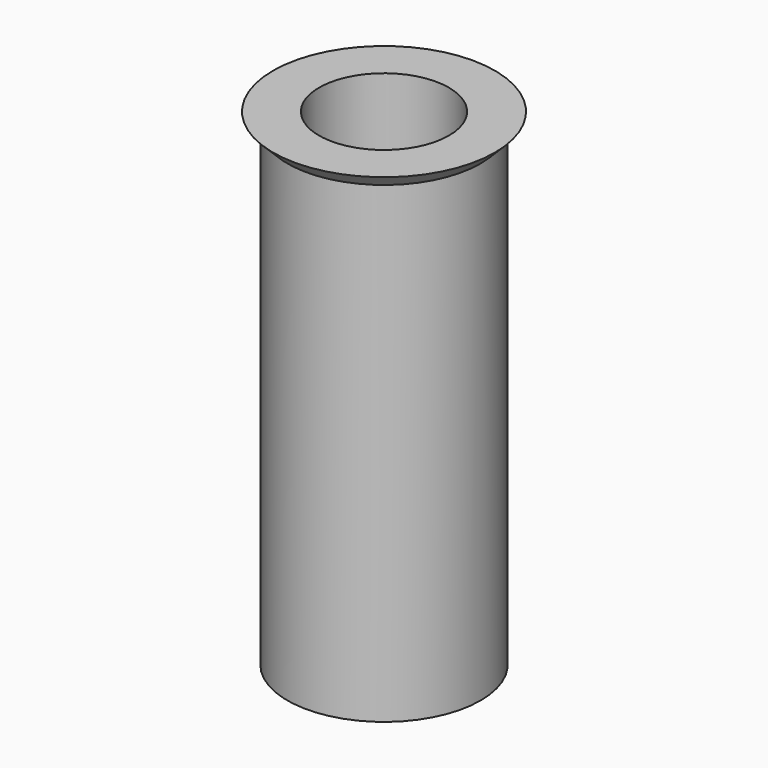
from build123d import *

# Parameters (mm, degrees)
F0_R        = 8.925
F1_DEPTH    = 45
F2_R        = 6
F3_DEPTH    = 40
F4_R        = 10.25
F4_R_2      = 8.925
F5_DEPTH    = 1.5
F6_S5_R     = 8.925
F6_T6_DEPTH = 16


# Not quite as in the source:
# - a fillet or chamfer that OpenCascade refuses, or shapes differently, is made with other operations: its cross-section is extruded or revolved along the edge and cut away or added


with BuildPart() as f1:
    # F0 (on Top) → F1 (new body)
    with BuildSketch(Plane.XY):
        Circle(F0_R)
    extrude(amount=F1_DEPTH)

    # F2 (on face) → F3 (cut)
    with BuildSketch(Plane.XY.offset(45)):
        Circle(F2_R)
    extrude(amount=-F3_DEPTH, mode=Mode.SUBTRACT)

    # F4 (on face) → F5 (join)
    with BuildSketch(Plane.XY.offset(45)):
        Circle(F4_R)
        Circle(F4_R_2, mode=Mode.SUBTRACT)
    extrude(amount=-F5_DEPTH)

    # F6: chamfer of 1.5 on 1 edges, made by hand


with BuildPart() as f6_tool2:
    # F6_s3 → F6_t4 (revolve)
    with BuildSketch(Plane.XZ):
        Polygon((8.75, 43.5), (10.25, 45), (10.25, 43.5), align=None)
    revolve(axis=Axis((0, 0, 43.5), (0, 0, 1)))

    # F6_s5 → F6_t6 (cut, symmetric)
    with BuildSketch(Plane.XY.offset(44.2)):
        Circle(F6_S5_R)
    extrude(amount=F6_T6_DEPTH, both=True, mode=Mode.SUBTRACT)


with BuildPart() as f1_1:
    add(f1.part)

    # F6_t1: cut F6_tool2
    add(f6_tool2.part, mode=Mode.SUBTRACT)


solid = f1_1.part
